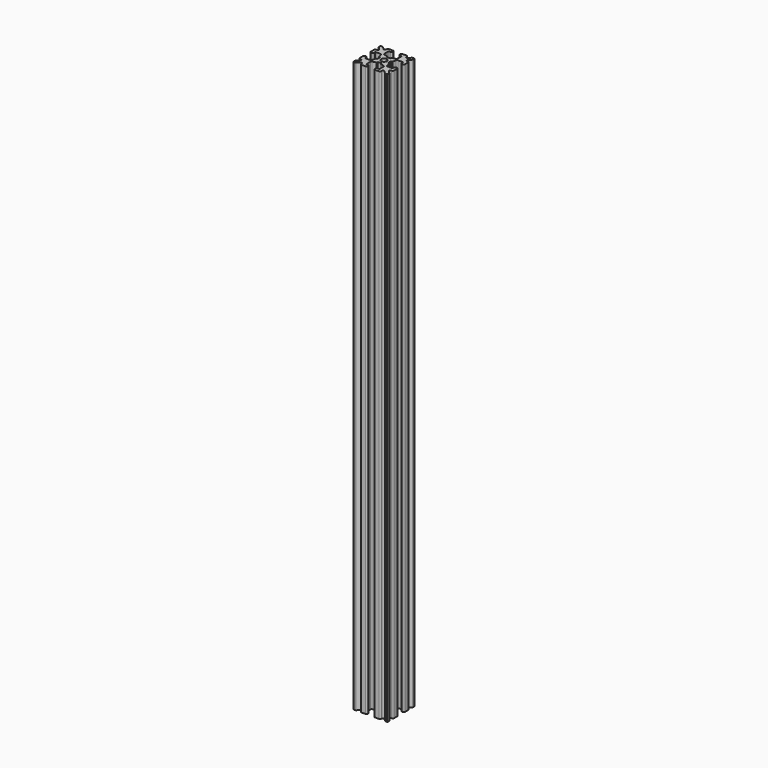
from build123d import *

# Parameters (mm, degrees)
F1_DEPTH = 250


# Not quite as in the source:
# - ends of sketch curves that miss each other by under 0.0002 mm in the source are joined


with BuildPart() as f1:
    # F0 (on Top) → F1 (new body)
    with BuildSketch(Plane.XY):
        with BuildLine():
            Line((-1.814515, 17.736209), (-2.91158, 17.736209))
            ThreePointArc((-2.91158, 17.736209), (-3.2776965235, 16.8523255235), (-4.16158, 16.486209))
            Line((-4.16158, 16.486209), (-4.16158, 15.389144))
            Line((-4.16158, 15.389144), (-3.53608, 15.389144))
            ThreePointArc((-3.53608, 15.389144), (-3.3946586438, 15.3305653562), (-3.33608, 15.189144))
            Line((-3.33608, 15.189144), (-3.33608, 14.961318))
            ThreePointArc((-3.33608, 14.961318), (-3.2922023866, 14.8363147984), (-3.1798219959, 14.7661600184))
            Line((-3.1798219959, 14.7661600184), (-1.652224, 14.423767))
            ThreePointArc((-1.652224, 14.423767), (-1.3712737286, 14.2483796232), (-1.26158, 13.935872))
            Line((-1.26158, 13.935872), (-1.26158, 11.836209))
            ThreePointArc((-1.26158, 11.836209), (-1.3201586438, 11.6947876438), (-1.46158, 11.636209))
            Line((-1.46158, 11.636209), (-2.06158, 11.636209))
            ThreePointArc((-2.06158, 11.636209), (-2.4151333906, 11.4897623906), (-2.56158, 11.136209))
            Line((-2.56158, 11.136209), (-2.56158, 10.736209))
            ThreePointArc((-2.56158, 10.736209), (-2.4151333906, 10.3826556094), (-2.06158, 10.236209))
            Line((-2.06158, 10.236209), (-0.26158, 10.236209))
            ThreePointArc((-0.26158, 10.236209), (0.0919733906, 10.3826556094), (0.23842, 10.736209))
            Line((0.23842, 10.736209), (0.23842, 11.068442))
            ThreePointArc((0.23842, 11.068442), (0.5470786105, 11.5303819016), (1.0919738906, 11.4219948906))
            Line((1.0919738906, 11.4219948906), (2.131313, 10.382656))
            ThreePointArc((2.131313, 10.382656), (2.2935249572, 10.274269369), (2.484867, 10.236209))
            Line((2.484867, 10.236209), (3.08842, 10.236209))
            ThreePointArc((3.08842, 10.236209), (3.2651966953, 10.3094323047), (3.33842, 10.486209))
            Line((3.33842, 10.486209), (3.33842, 11.089762))
            ThreePointArc((3.33842, 11.089762), (3.3003597663, 11.2811037162), (3.1919733906, 11.4433153906))
            Line((3.1919733906, 11.4433153906), (2.152634, 12.482656))
            ThreePointArc((2.152634, 12.482656), (2.0442472337, 13.0275507162), (2.506187, 13.336209))
            Line((2.506187, 13.336209), (2.83842, 13.336209))
            ThreePointArc((2.83842, 13.336209), (3.1919733906, 13.4826556094), (3.33842, 13.836209))
            Line((3.33842, 13.836209), (3.33842, 15.636209))
            ThreePointArc((3.33842, 15.636209), (3.1919733906, 15.9897623906), (2.83842, 16.136209))
            Line((2.83842, 16.136209), (2.43842, 16.136209))
            ThreePointArc((2.43842, 16.136209), (2.0848666094, 15.9897623906), (1.93842, 15.636209))
            Line((1.93842, 15.636209), (1.93842, 15.036209))
            ThreePointArc((1.93842, 15.036209), (1.8798413562, 14.8947876438), (1.73842, 14.836209))
            Line((1.73842, 14.836209), (-0.361243, 14.836209))
            ThreePointArc((-0.361243, 14.836209), (-0.6737506232, 14.9459027286), (-0.8491377407, 15.2268530581))
            Line((-0.8491377407, 15.2268530581), (-1.191531, 16.754451))
            ThreePointArc((-1.191531, 16.754451), (-1.2616857984, 16.8668313866), (-1.386689, 16.910709))
            Line((-1.386689, 16.910709), (-1.614515, 16.910709))
            ThreePointArc((-1.614515, 16.910709), (-1.7559363562, 16.9692876438), (-1.814515, 17.110709))
            Line((-1.814515, 17.110709), (-1.814515, 17.736209))
        make_face()
        with BuildLine():
            ThreePointArc((-4.16158, 18.986209), (-3.2776965235, 18.6200924765), (-2.91158, 17.736209))
            Line((-2.91158, 17.736209), (-1.814515, 17.736209))
            Line((-1.814515, 17.736209), (-1.814515, 18.361709))
            ThreePointArc((-1.814515, 18.361709), (-1.7559363562, 18.5031303562), (-1.614515, 18.561709))
            Line((-1.614515, 18.561709), (-1.386689, 18.561709))
            ThreePointArc((-1.386689, 18.561709), (-1.2616857984, 18.6055866134), (-1.1915310184, 18.7179670041))
            Line((-1.1915310184, 18.7179670041), (-0.849138, 20.245565))
            ThreePointArc((-0.849138, 20.245565), (-0.6737506232, 20.5265152714), (-0.361243, 20.636209))
            Line((-0.361243, 20.636209), (1.73842, 20.636209))
            ThreePointArc((1.73842, 20.636209), (1.8798413562, 20.5776303562), (1.93842, 20.436209))
            Line((1.93842, 20.436209), (1.93842, 19.836209))
            ThreePointArc((1.93842, 19.836209), (2.0848666094, 19.4826556094), (2.43842, 19.336209))
            Line((2.43842, 19.336209), (2.83842, 19.336209))
            ThreePointArc((2.83842, 19.336209), (3.1919733906, 19.4826556094), (3.33842, 19.836209))
            Line((3.33842, 19.836209), (3.33842, 21.636209))
            ThreePointArc((3.33842, 21.636209), (3.1919733906, 21.9897623906), (2.83842, 22.136209))
            Line((2.83842, 22.136209), (2.506187, 22.136209))
            ThreePointArc((2.506187, 22.136209), (2.0442472337, 22.4448672838), (2.1526336094, 22.9897623906))
            Line((2.1526336094, 22.9897623906), (3.191974, 24.029102))
            ThreePointArc((3.191974, 24.029102), (3.3003597663, 24.1913142838), (3.33842, 24.382656))
            Line((3.33842, 24.382656), (3.33842, 24.986209))
            ThreePointArc((3.33842, 24.986209), (3.2651966953, 25.1629856953), (3.08842, 25.236209))
            Line((3.08842, 25.236209), (2.484867, 25.236209))
            ThreePointArc((2.484867, 25.236209), (2.2935249572, 25.198148631), (2.1313131094, 25.0897618906))
            Line((2.1313131094, 25.0897618906), (1.091974, 24.050423))
            ThreePointArc((1.091974, 24.050423), (0.5470786105, 23.9420360984), (0.23842, 24.403976))
            Line((0.23842, 24.403976), (0.23842, 24.736209))
            ThreePointArc((0.23842, 24.736209), (0.0919733906, 25.0897623906), (-0.26158, 25.236209))
            Line((-0.26158, 25.236209), (-2.06158, 25.236209))
            ThreePointArc((-2.06158, 25.236209), (-2.4151333906, 25.0897623906), (-2.56158, 24.736209))
            Line((-2.56158, 24.736209), (-2.56158, 24.336209))
            ThreePointArc((-2.56158, 24.336209), (-2.4151333906, 23.9826556094), (-2.06158, 23.836209))
            Line((-2.06158, 23.836209), (-1.46158, 23.836209))
            ThreePointArc((-1.46158, 23.836209), (-1.3201586438, 23.7776303562), (-1.26158, 23.636209))
            Line((-1.26158, 23.636209), (-1.26158, 21.536546))
            ThreePointArc((-1.26158, 21.536546), (-1.3712737286, 21.2240383768), (-1.6522240581, 21.0486512593))
            Line((-1.6522240581, 21.0486512593), (-3.179822, 20.706258))
            ThreePointArc((-3.179822, 20.706258), (-3.2922023866, 20.6361032016), (-3.33608, 20.5111))
            Line((-3.33608, 20.5111), (-3.33608, 20.283274))
            ThreePointArc((-3.33608, 20.283274), (-3.3946586438, 20.1418526438), (-3.53608, 20.083274))
            Line((-3.53608, 20.083274), (-4.16158, 20.083274))
            Line((-4.16158, 20.083274), (-4.16158, 18.986209))
        make_face()
        with BuildLine():
            ThreePointArc((-5.41158, 17.736209), (-5.0454634765, 18.6200924765), (-4.16158, 18.986209))
            Line((-4.16158, 18.986209), (-4.16158, 20.083274))
            Line((-4.16158, 20.083274), (-4.78708, 20.083274))
            ThreePointArc((-4.78708, 20.083274), (-4.9285013562, 20.1418526438), (-4.98708, 20.283274))
            Line((-4.98708, 20.283274), (-4.98708, 20.5111))
            ThreePointArc((-4.98708, 20.5111), (-5.0309576134, 20.6361032016), (-5.1433380041, 20.7062579816))
            Line((-5.1433380041, 20.7062579816), (-6.670936, 21.048651))
            ThreePointArc((-6.670936, 21.048651), (-6.9518862714, 21.2240383768), (-7.06158, 21.536546))
            Line((-7.06158, 21.536546), (-7.06158, 23.636209))
            ThreePointArc((-7.06158, 23.636209), (-7.0030013562, 23.7776303562), (-6.86158, 23.836209))
            Line((-6.86158, 23.836209), (-6.26158, 23.836209))
            ThreePointArc((-6.26158, 23.836209), (-5.9080266094, 23.9826556094), (-5.76158, 24.336209))
            Line((-5.76158, 24.336209), (-5.76158, 24.736209))
            ThreePointArc((-5.76158, 24.736209), (-5.9080266094, 25.0897623906), (-6.26158, 25.236209))
            Line((-6.26158, 25.236209), (-8.06158, 25.236209))
            ThreePointArc((-8.06158, 25.236209), (-8.4151333906, 25.0897623906), (-8.56158, 24.736209))
            Line((-8.56158, 24.736209), (-8.56158, 24.403976))
            ThreePointArc((-8.56158, 24.403976), (-8.8702382838, 23.9420362337), (-9.4151333906, 24.0504226094))
            Line((-9.4151333906, 24.0504226094), (-10.454473, 25.089762))
            ThreePointArc((-10.454473, 25.089762), (-10.6166842838, 25.1981487663), (-10.808026, 25.236209))
            Line((-10.808026, 25.236209), (-11.41158, 25.236209))
            ThreePointArc((-11.41158, 25.236209), (-11.5883566953, 25.1629856953), (-11.66158, 24.986209))
            Line((-11.66158, 24.986209), (-11.66158, 24.382656))
            ThreePointArc((-11.66158, 24.382656), (-11.623519631, 24.1913139572), (-11.5151328906, 24.0291021094))
            Line((-11.5151328906, 24.0291021094), (-10.475793, 22.989762))
            ThreePointArc((-10.475793, 22.989762), (-10.367407369, 22.4448669572), (-10.829347, 22.136209))
            Line((-10.829347, 22.136209), (-11.16158, 22.136209))
            ThreePointArc((-11.16158, 22.136209), (-11.5151333906, 21.9897623906), (-11.66158, 21.636209))
            Line((-11.66158, 21.636209), (-11.66158, 19.836209))
            ThreePointArc((-11.66158, 19.836209), (-11.5151333906, 19.4826556094), (-11.16158, 19.336209))
            Line((-11.16158, 19.336209), (-10.76158, 19.336209))
            ThreePointArc((-10.76158, 19.336209), (-10.4080266094, 19.4826556094), (-10.26158, 19.836209))
            Line((-10.26158, 19.836209), (-10.26158, 20.436209))
            ThreePointArc((-10.26158, 20.436209), (-10.2030013562, 20.5776303562), (-10.06158, 20.636209))
            Line((-10.06158, 20.636209), (-7.961916, 20.636209))
            ThreePointArc((-7.961916, 20.636209), (-7.6494084622, 20.5265153397), (-7.4740213072, 20.2455651553))
            Line((-7.4740213072, 20.2455651553), (-7.131629, 18.717967))
            ThreePointArc((-7.131629, 18.717967), (-7.0614742016, 18.6055866134), (-6.936471, 18.561709))
            Line((-6.936471, 18.561709), (-6.708644, 18.561709))
            ThreePointArc((-6.708644, 18.561709), (-6.5672226438, 18.5031303562), (-6.508644, 18.361709))
            Line((-6.508644, 18.361709), (-6.508644, 17.736209))
            Line((-6.508644, 17.736209), (-5.41158, 17.736209))
        make_face()
        with BuildLine():
            Line((-4.16158, 15.389144), (-4.16158, 16.486209))
            ThreePointArc((-4.16158, 16.486209), (-5.0454634765, 16.8523255235), (-5.41158, 17.736209))
            Line((-5.41158, 17.736209), (-6.508644, 17.736209))
            Line((-6.508644, 17.736209), (-6.508644, 17.110709))
            ThreePointArc((-6.508644, 17.110709), (-6.5672226438, 16.9692876438), (-6.708644, 16.910709))
            Line((-6.708644, 16.910709), (-6.936471, 16.910709))
            ThreePointArc((-6.936471, 16.910709), (-7.0614742016, 16.8668313866), (-7.1316289816, 16.7544509959))
            Line((-7.1316289816, 16.7544509959), (-7.474022, 15.226853))
            ThreePointArc((-7.474022, 15.226853), (-7.6494084622, 14.9459026603), (-7.961916, 14.836209))
            Line((-7.961916, 14.836209), (-10.06158, 14.836209))
            ThreePointArc((-10.06158, 14.836209), (-10.2030013562, 14.8947876438), (-10.26158, 15.036209))
            Line((-10.26158, 15.036209), (-10.26158, 15.636209))
            ThreePointArc((-10.26158, 15.636209), (-10.4080266094, 15.9897623906), (-10.76158, 16.136209))
            Line((-10.76158, 16.136209), (-11.16158, 16.136209))
            ThreePointArc((-11.16158, 16.136209), (-11.5151333906, 15.9897623906), (-11.66158, 15.636209))
            Line((-11.66158, 15.636209), (-11.66158, 13.836209))
            ThreePointArc((-11.66158, 13.836209), (-11.5151333906, 13.4826556094), (-11.16158, 13.336209))
            Line((-11.16158, 13.336209), (-10.829347, 13.336209))
            ThreePointArc((-10.829347, 13.336209), (-10.367407369, 13.0275510428), (-10.4757931094, 12.4826561094))
            Line((-10.4757931094, 12.4826561094), (-11.515133, 11.443316))
            ThreePointArc((-11.515133, 11.443316), (-11.623519631, 11.2811040428), (-11.66158, 11.089762))
            Line((-11.66158, 11.089762), (-11.66158, 10.486209))
            ThreePointArc((-11.66158, 10.486209), (-11.5883566953, 10.3094323047), (-11.41158, 10.236209))
            Line((-11.41158, 10.236209), (-10.808026, 10.236209))
            ThreePointArc((-10.808026, 10.236209), (-10.6166842838, 10.2742692337), (-10.4544726094, 10.3826556094))
            Line((-10.4544726094, 10.3826556094), (-9.415133, 11.421995))
            ThreePointArc((-9.415133, 11.421995), (-8.8702382838, 11.5303817663), (-8.56158, 11.068442))
            Line((-8.56158, 11.068442), (-8.56158, 10.736209))
            ThreePointArc((-8.56158, 10.736209), (-8.4151333906, 10.3826556094), (-8.06158, 10.236209))
            Line((-8.06158, 10.236209), (-6.26158, 10.236209))
            ThreePointArc((-6.26158, 10.236209), (-5.9080266094, 10.3826556094), (-5.76158, 10.736209))
            Line((-5.76158, 10.736209), (-5.76158, 11.136209))
            ThreePointArc((-5.76158, 11.136209), (-5.9080266094, 11.4897623906), (-6.26158, 11.636209))
            Line((-6.26158, 11.636209), (-6.86158, 11.636209))
            ThreePointArc((-6.86158, 11.636209), (-7.0030013562, 11.6947876438), (-7.06158, 11.836209))
            Line((-7.06158, 11.836209), (-7.06158, 13.935872))
            ThreePointArc((-7.06158, 13.935872), (-6.9518862714, 14.2483796232), (-6.6709359419, 14.4237667407))
            Line((-6.6709359419, 14.4237667407), (-5.143338, 14.76616))
            ThreePointArc((-5.143338, 14.76616), (-5.0309576134, 14.8363147984), (-4.98708, 14.961318))
            Line((-4.98708, 14.961318), (-4.98708, 15.189144))
            ThreePointArc((-4.98708, 15.189144), (-4.9285013562, 15.3305653562), (-4.78708, 15.389144))
            Line((-4.78708, 15.389144), (-4.16158, 15.389144))
        make_face()
    extrude(amount=F1_DEPTH)


solid = f1.part
